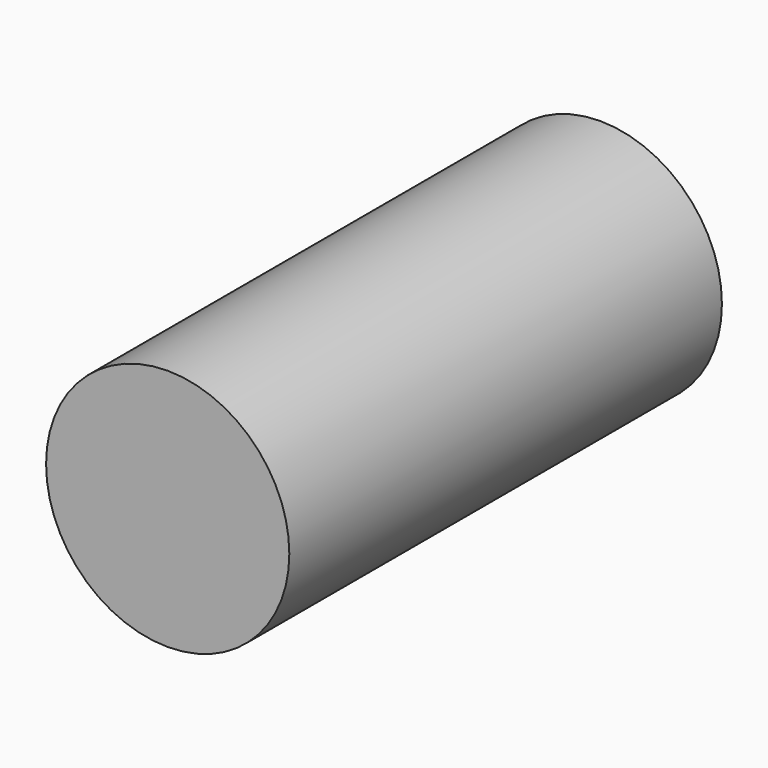
from build123d import *

# Parameters (mm, degrees)
F0_R     = 44.8628233992
F1_DEPTH = 199.47085


# Not quite as in the source:
# - the program builds the solid bodies; features that only make, move or delete a surface that nothing else refers to are left out


with BuildPart() as f1:
    # F0 (on Front) → F1 (new body)
    with BuildSketch(Plane.XZ):
        Circle(F0_R)
    extrude(amount=F1_DEPTH)


solid = f1.part
